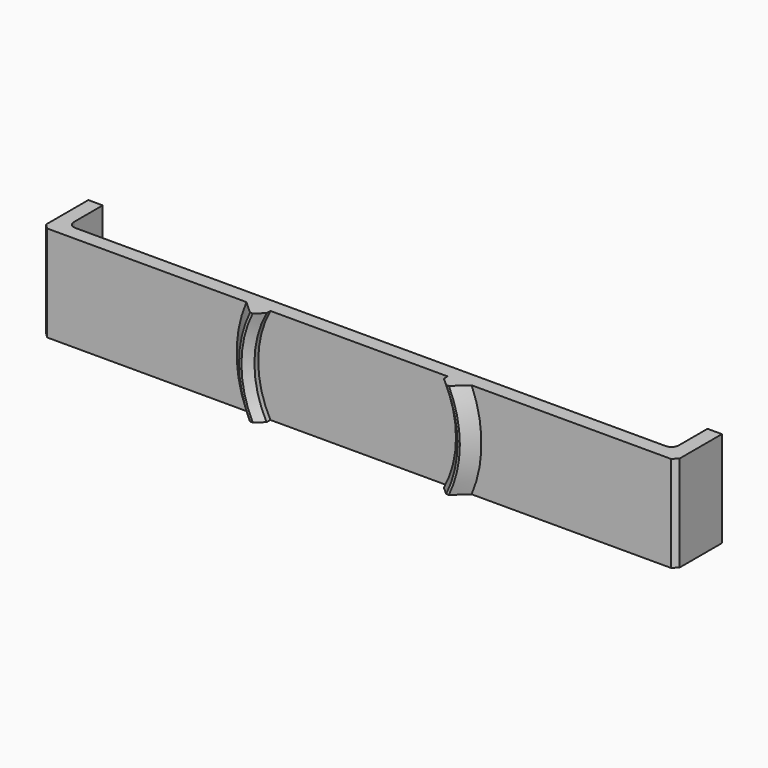
from build123d import *

# Parameters (mm, degrees)
F1_DEPTH = 10
F3_DEPTH = 2.5
F4_SIZE  = 1.5
F5_SIZE  = 2.49999
F6_SIZE  = 1
F7_R     = 1.5


# Not quite as in the source:
# - a fillet or chamfer is up to 0.001 mm smaller than in the source, because OpenCascade refuses the exact size


with BuildPart() as f1:
    # F0 (on Top) → F1 (new body, symmetric)
    with BuildSketch(Plane.XY):
        Polygon((63, 0), (-63, 0), (-63, 9), (-66, 9), (-66, -3), (66, -3), (66, 9), (63, 9), align=None)
    extrude(amount=F1_DEPTH, both=True)

    # F2 (on face) → F3 (join)
    with BuildSketch(Plane.XZ.offset(3)):
        with BuildLine():
            ThreePointArc((-18.4661853126, -10), (-21, 0), (-18.4661853126, 10))
            Line((-18.4661853126, 10), (-20.7123151772, 10))
            ThreePointArc((-20.7123151772, 10), (-23, 0), (-20.7123151772, -10))
            Line((-20.7123151772, -10), (-18.4661853126, -10))
        make_face()
        with BuildLine():
            Line((20.7123151772, 10), (18.4661853126, 10))
            ThreePointArc((18.4661853126, 10), (21, 0), (18.4661853126, -10))
            Line((18.4661853126, -10), (20.7123151772, -10))
            ThreePointArc((20.7123151772, -10), (23, 0), (20.7123151772, 10))
        make_face()
    extrude(amount=F3_DEPTH)

    # F4
    f4_edges = [f1.edges().sort_by_distance(p)[0] for p in [
        (-21, -5.5, 0),
        (21, -5.5, 0),
    ]]
    chamfer(f4_edges, length=F4_SIZE)

    # F5 (size 2.5 in the source; OpenCascade refuses exactly that, so slightly less here)
    f5_edges = [f1.edges().sort_by_distance(p)[0] for p in [
        (-23, -3, 0),
        (23, -3, 0),
    ]]
    chamfer(f5_edges, length=F5_SIZE)

    # F6
    f6_edges = [f1.edges().sort_by_distance(p)[0] for p in [
        (-66, -3, 0),
        (66, -3, 0),
    ]]
    chamfer(f6_edges, length=F6_SIZE)

    # F7
    f7_edges = [f1.edges().sort_by_distance(p)[0] for p in [
        (63, 0, 0),
        (-63, 0, 0),
    ]]
    fillet(f7_edges, radius=F7_R)


solid = f1.part
